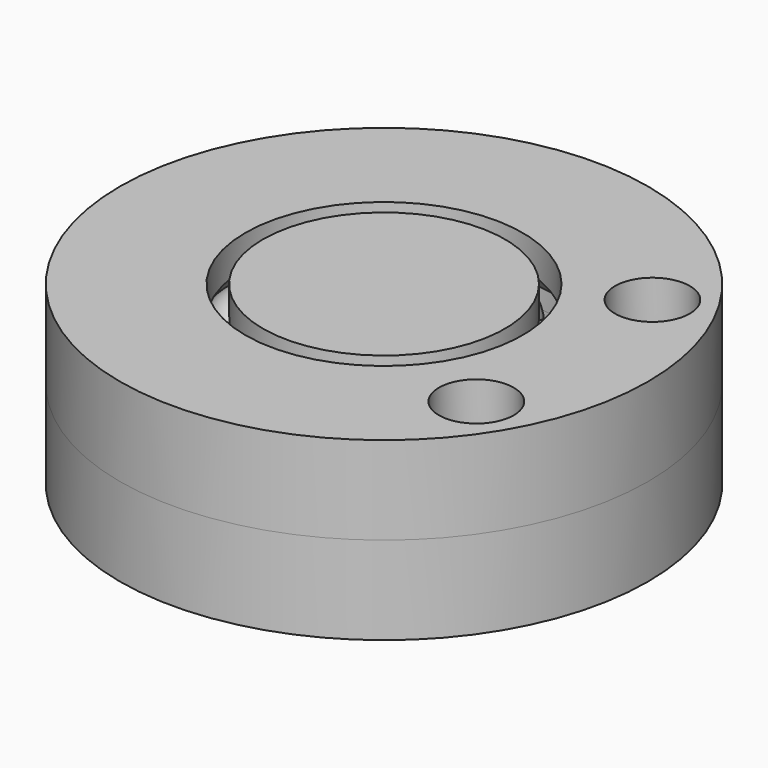
from build123d import *

# Parameters (mm, degrees)
F6_COUNT  = 8
F6_ANGLE  = 315
F7_R      = 4.25
F7_R_2    = 1.925
F8_DEPTH  = 5
F9_DEPTH  = 15
F10_R     = 1.925
F11_DEPTH = 5
F12_DEPTH = 5
F13_R     = 4.25
F14_DEPTH = 5
F15_R     = 4.25
F16_DEPTH = 5


# Not quite as in the source:
# - a feature names something its author has since deleted; it is built from what else it names


with BuildPart() as f1:
    # F0 (on Front) → F1 (revolve)
    with BuildSketch(Plane.XZ):
        Polygon((-20, 0), (-30, 0), (-30, -10), (-15.75, -10), (-15.75, -6.4246212025), (-20, -2.1746212025), align=None)
    revolve(axis=Axis((0, 0, -5), (0, 0, -1)))

    # F10 (on Top) → F11 (cut)
    with BuildSketch(Plane.XY):
        with Locations((20.4878012485, 12.5)):
            Circle(F10_R)
        with Locations((20.4878012485, -12.5)):
            Circle(F10_R)
        with Locations((-20.4878012485, -12.5)):
            Circle(F10_R)
        with Locations((-20.4878012485, 12.5)):
            Circle(F10_R)
    extrude(amount=-F11_DEPTH, mode=Mode.SUBTRACT)

    # F15 (on face) → F16 (cut)
    with BuildSketch(Plane(origin=(0, 0, -10), x_dir=(1, 0, 0), z_dir=(0, 0, -1))):
        with Locations((-20.4878012485, 12.5)):
            Circle(F15_R)
        with Locations((-20.4878012485, -12.5)):
            Circle(F15_R)
    extrude(amount=-F16_DEPTH, mode=Mode.SUBTRACT)


with BuildPart() as f2:
    # F0 (on Front) → F2 (revolve)
    with BuildSketch(Plane.XZ):
        Polygon((-30, 10), (-30, 0), (-20, 0), (-20, 2.1746212025), (-15.75, 6.4246212025), (-15.75, 10), align=None)
    revolve(axis=Axis((0, 0, 0), (0, 0, -1)))

    # F10 (on Top) → F12 (cut)
    with BuildSketch(Plane.XY):
        with Locations((20.4878012485, -12.5)):
            Circle(F10_R)
        with Locations((20.4878012485, 12.5)):
            Circle(F10_R)
        with Locations((-20.4878012485, -12.5)):
            Circle(F10_R)
        with Locations((-20.4878012485, 12.5)):
            Circle(F10_R)
    extrude(amount=F12_DEPTH, mode=Mode.SUBTRACT)

    # F13 (on face) → F14 (cut)
    with BuildSketch(Plane.XY.offset(10)):
        with Locations((20.4878012485, -12.5)):
            Circle(F13_R)
        with Locations((20.4878012485, 12.5)):
            Circle(F13_R)
    extrude(amount=-F14_DEPTH, mode=Mode.SUBTRACT)


with BuildPart() as f3:
    # F0 (on Front) → F3 (revolve)
    with BuildSketch(Plane.XZ):
        Polygon((-13.75, -6.4246212025), (-13.75, -10), (0, -10), (0, 0), (-7.3253787975, 0), align=None)
    revolve(axis=Axis((0, 0, -5), (0, 0, -1)))

    # F7 (on face) → F8 (cut)
    with BuildSketch(Plane(origin=(0, 0, -10), x_dir=(1, 0, 0), z_dir=(0, 0, -1))):
        Circle(F7_R)
        Circle(F7_R_2, mode=Mode.SUBTRACT)
        Circle(F7_R_2)
    extrude(amount=-F8_DEPTH, mode=Mode.SUBTRACT)


with BuildPart() as f4:
    # F0 (on Front) → F4 (revolve)
    with BuildSketch(Plane.XZ):
        Polygon((-13.75, 6.4246212025), (-7.3253787975, 0), (0, 0), (0, 10), (-13.75, 10), align=None)
    revolve(axis=Axis((0, 0, 5), (0, 0, -1)))


with BuildPart() as f5:
    # F0 (on Front) → F5 (revolve)
    with BuildSketch(Plane.XZ):
        with BuildLine():
            Line((-14.75, -5), (-14.75, 5))
            ThreePointArc((-14.75, 5), (-19.75, 0), (-14.75, -5))
        make_face()
    revolve(axis=Axis((-14.75, 0, 0), (0, 0, -1)))


with BuildPart() as f6_1:
    # F6: instance of F5
    add(f5.part.rotate(Axis((0, 0, 5), (0, 0, -1)), 1 * F6_ANGLE / (F6_COUNT - 1)))


with BuildPart() as f6_2:
    # F6: instance of F5
    add(f5.part.rotate(Axis((0, 0, 5), (0, 0, -1)), 2 * F6_ANGLE / (F6_COUNT - 1)))


with BuildPart() as f6_3:
    # F6: instance of F5
    add(f5.part.rotate(Axis((0, 0, 5), (0, 0, -1)), 3 * F6_ANGLE / (F6_COUNT - 1)))


with BuildPart() as f6_4:
    # F6: instance of F5
    add(f5.part.rotate(Axis((0, 0, 5), (0, 0, -1)), 4 * F6_ANGLE / (F6_COUNT - 1)))


with BuildPart() as f6_5:
    # F6: instance of F5
    add(f5.part.rotate(Axis((0, 0, 5), (0, 0, -1)), 5 * F6_ANGLE / (F6_COUNT - 1)))


with BuildPart() as f6_6:
    # F6: instance of F5
    add(f5.part.rotate(Axis((0, 0, 5), (0, 0, -1)), 6 * F6_ANGLE / (F6_COUNT - 1)))


with BuildPart() as f6_7:
    # F6: instance of F5
    add(f5.part.rotate(Axis((0, 0, 5), (0, 0, -1)), 7 * F6_ANGLE / (F6_COUNT - 1)))


with BuildPart() as f9_tool:
    # F7 (on face) → F9 (new body)
    with BuildSketch(Plane(origin=(0, 0, -10), x_dir=(1, 0, 0), z_dir=(0, 0, -1))):
        Circle(F7_R_2)
    extrude(amount=-F9_DEPTH)


with BuildPart() as f3_1:
    add(f3.part)

    # F9: cut by f9_tool
    add(f9_tool.part, mode=Mode.SUBTRACT)


with BuildPart() as f4_1:
    add(f4.part)

    # F9: cut by f9_tool
    add(f9_tool.part, mode=Mode.SUBTRACT)


solid = Compound([f1.part, f2.part, f5.part, f6_1.part, f6_2.part, f6_3.part, f6_4.part, f6_5.part, f6_6.part, f6_7.part, f3_1.part, f4_1.part])
